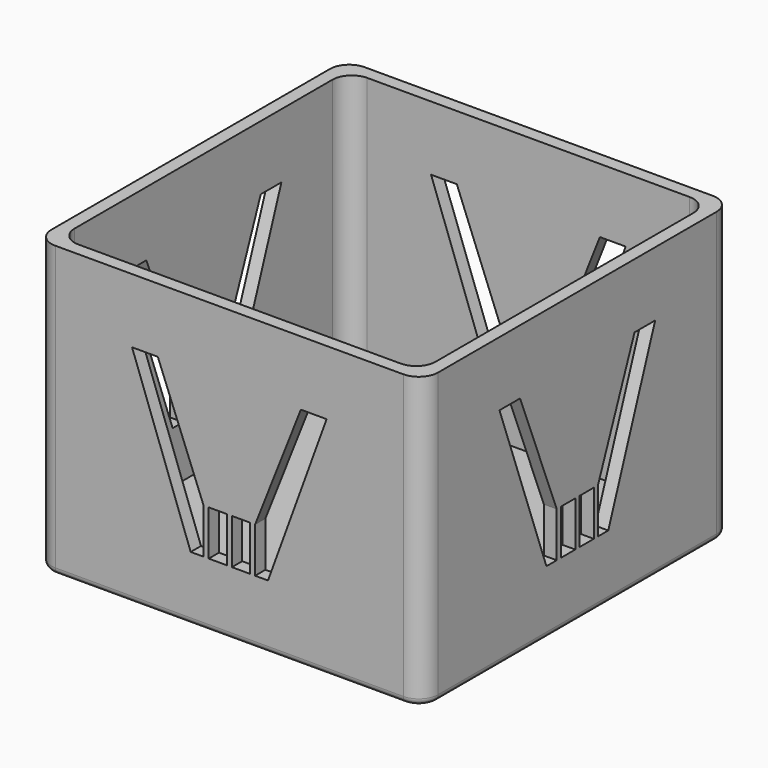
from build123d import *

# Parameters (mm, degrees)
F0_W     = 60
F0_H     = 60
F1_DEPTH = 45
F2_T     = -2
F3_W     = 2.8
F3_H     = 7
F4_DEPTH = 64.2
F5_W     = 2.8
F5_H     = 7
F6_DEPTH = 63.5
F8_DEPTH = 25
F9_R     = 3
F10_R    = 1


# Not quite as in the source:
# - a feature names something its author has since deleted; it is built from what else it names


with BuildPart() as f1:
    # F0 (on Top) → F1 (new body)
    with BuildSketch(Plane.XY):
        Rectangle(F0_W, F0_H)
    extrude(amount=F1_DEPTH)

    # F2
    f2_openings = [f1.faces().sort_by_distance(p)[0] for p in [
        (0, 0, 45),
    ]]
    offset(amount=F2_T, openings=f2_openings)

    # F3 (on face) → F4 (cut)
    with BuildSketch(Plane.XZ.offset(30)):
        Polygon((-15.0992558567, 35), (-6, 10), (-4, 10), (-4, 17), (-11.0992558567, 35), align=None)
        with Locations((-1.8, 13.5)):
            Rectangle(F3_W, F3_H)
        with Locations((1.8, 13.5)):
            Rectangle(F3_W, F3_H)
        Polygon((4, 17), (4, 10), (6, 10), (15.0992558567, 35), (11.0992558567, 35), align=None)
    extrude(amount=-F4_DEPTH, mode=Mode.SUBTRACT)

    # F5 (on face) → F6 (cut)
    with BuildSketch(Plane.YZ.offset(30)):
        Polygon((-15.0992558567, 35), (-6, 10), (-4, 10), (-4, 17), (-11.0992558567, 35), align=None)
        with Locations((-1.8, 13.5)):
            Rectangle(F5_W, F5_H)
        with Locations((1.8, 13.5)):
            Rectangle(F5_W, F5_H)
        Polygon((4, 17), (4, 10), (6, 10), (15.0992558567, 35), (11.0992558567, 35), align=None)
    extrude(amount=-F6_DEPTH, mode=Mode.SUBTRACT)

    # F7 (on face) → F8 (cut)
    with BuildSketch(Plane(origin=(0, 0, 0), x_dir=(1, 0, 0), z_dir=(0, 0, -1))):
        with BuildLine():
            Line((0.9656854249, 0.4), (9.9919967974, 0.4))
            ThreePointArc((9.9919967974, 0.4), (9.2387953251, 3.8268343237), (7.3482514055, 6.7825659806))
            Line((7.3482514055, 6.7825659806), (0.9656854249, 0.4))
        make_face()
        with BuildLine():
            ThreePointArc((7.3482514055, -6.7825659806), (9.2387953251, -3.8268343237), (9.9919967974, -0.4))
            Line((9.9919967974, -0.4), (0.9656854249, -0.4))
            Line((0.9656854249, -0.4), (7.3482514055, -6.7825659806))
        make_face()
        with BuildLine():
            Line((0.4, 0.9656854249), (6.7825659806, 7.3482514055))
            ThreePointArc((6.7825659806, 7.3482514055), (3.8268343237, 9.2387953251), (0.4, 9.9919967974))
            Line((0.4, 9.9919967974), (0.4, 0.9656854249))
        make_face()
        with BuildLine():
            ThreePointArc((0.4, -9.9919967974), (3.8268343237, -9.2387953251), (6.7825659806, -7.3482514055))
            Line((6.7825659806, -7.3482514055), (0.4, -0.9656854249))
            Line((0.4, -0.9656854249), (0.4, -9.9919967974))
        make_face()
        with BuildLine():
            Line((-6.7825659806, 7.3482514055), (-0.4, 0.9656854249))
            Line((-0.4, 0.9656854249), (-0.4, 9.9919967974))
            ThreePointArc((-0.4, 9.9919967974), (-3.8268343237, 9.2387953251), (-6.7825659806, 7.3482514055))
        make_face()
        with BuildLine():
            Line((-0.4, -9.9919967974), (-0.4, -0.9656854249))
            Line((-0.4, -0.9656854249), (-6.7825659806, -7.3482514055))
            ThreePointArc((-6.7825659806, -7.3482514055), (-3.8268343237, -9.2387953251), (-0.4, -9.9919967974))
        make_face()
        with BuildLine():
            Line((-7.3482514055, -6.7825659806), (-0.9656854249, -0.4))
            Line((-0.9656854249, -0.4), (-9.9919967974, -0.4))
            ThreePointArc((-9.9919967974, -0.4), (-9.2387953251, -3.8268343237), (-7.3482514055, -6.7825659806))
        make_face()
        with BuildLine():
            Line((-9.9919967974, 0.4), (-0.9656854249, 0.4))
            Line((-0.9656854249, 0.4), (-7.3482514055, 6.7825659806))
            ThreePointArc((-7.3482514055, 6.7825659806), (-9.2387953251, 3.8268343237), (-9.9919967974, 0.4))
        make_face()
    extrude(amount=-F8_DEPTH, mode=Mode.SUBTRACT)

    # F9
    f9_edges = [f1.edges().sort_by_distance(p)[0] for p in [
        (-30, -30, 22.5),
        (30, -30, 22.5),
        (30, 30, 22.5),
        (-30, 30, 22.5),
        (-28, -28, 23.5),
        (28, -28, 23.5),
        (28, 28, 23.5),
        (-28, 28, 23.5),
    ]]
    fillet(f9_edges, radius=F9_R)

    # F10
    f10_edges = [f1.edges().sort_by_distance(p)[0] for p in [
        (0, -30, 0),
        (-30, 0, 0),
        (30, 0, 0),
        (0, 30, 0),
        (29.12132, 29.12132, 0),
        (-29.12132, 29.12132, 0),
        (29.12132, -29.12132, 0),
        (-29.12132, -29.12132, 0),
    ]]
    fillet(f10_edges, radius=F10_R)


solid = f1.part
